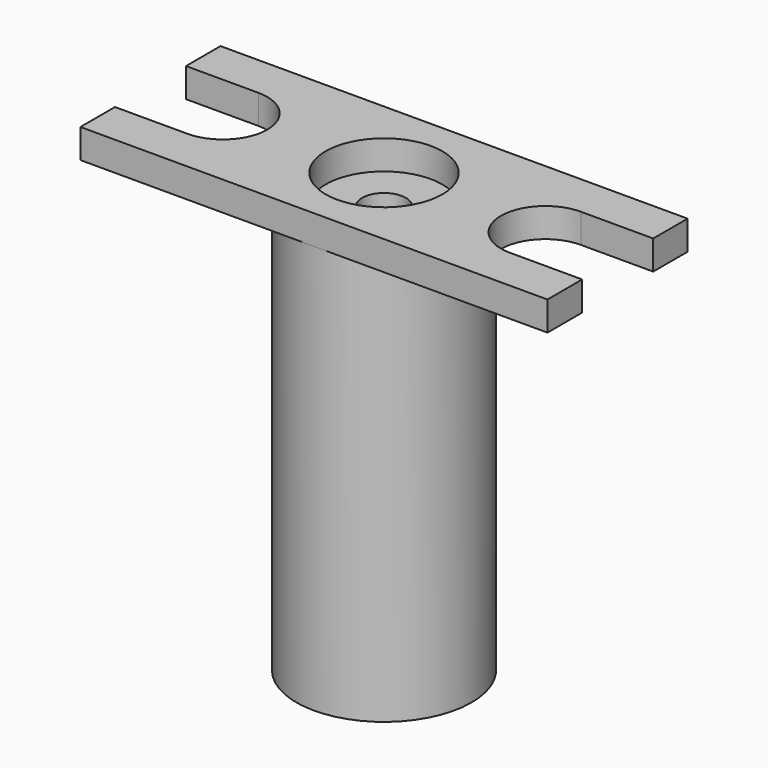
from build123d import *

# Parameters (mm, degrees)
F0_R        = 12.7
F1_DEPTH    = 6.35
F2_R        = 12.7
F3_DEPTH    = 63.5
F3_FACE_R   = 19.05
F3_FACE_R_2 = 12.7
F4_R        = 19.05
F4_R_2      = 4.7625
F5_DEPTH    = 25.4


with BuildPart() as f1:
    # F0 (on Top) → F1 (new body)
    with BuildSketch(Plane.XY):
        with BuildLine():
            Line((0, 9.398), (0, 0))
            Line((0, 0), (101.6, 0))
            Line((101.6, 0), (101.6, 9.4413837329))
            Line((101.6, 9.4413837329), (85.851973152, 9.4413837329))
            ThreePointArc((85.851973152, 9.4413837329), (76.199973152, 19.0933837329), (85.851973152, 28.7453837329))
            Line((85.851973152, 28.7453837329), (101.6, 28.7453837329))
            Line((101.6, 28.7453837329), (101.6, 38.1))
            Line((101.6, 38.1), (50.7999907375, 38.1))
            Line((50.7999907375, 38.1), (-1.85251e-05, 38.1))
            Line((-1.85251e-05, 38.1), (-1.85251e-05, 28.702))
            Line((-1.85251e-05, 28.702), (15.748, 28.702))
            ThreePointArc((15.748, 28.702), (25.4, 19.05), (15.748, 9.398))
            Line((15.748, 9.398), (0, 9.398))
        make_face()
        with Locations((50.8, 19.05)):
            Circle(F0_R, mode=Mode.SUBTRACT)
    extrude(amount=F1_DEPTH)

    # F2 (on face) → F3 (join)
    with BuildSketch(Plane(origin=(0, 0, 0), x_dir=(1, 0, 0), z_dir=(0, 0, -1))):
        with BuildLine():
            ThreePointArc((50.8, -38.1), (64.2703841816, -32.5203841816), (69.85, -19.05))
            ThreePointArc((69.85, -19.05), (64.2703841816, -5.5796158184), (50.8, 0))
            ThreePointArc((50.8, 0), (31.75, -19.05), (50.8, -38.1))
        make_face()
        with Locations((50.8, -19.05)):
            Circle(F2_R, mode=Mode.SUBTRACT)
    extrude(amount=F3_DEPTH)

    # F3_face (on face) + F4 (on Top) → F5 (join)
    with BuildSketch(Plane(origin=(50.8, 19.05, -63.5), x_dir=(1, 0, 0), z_dir=(0, 0, -1))):
        Circle(F3_FACE_R)
        Circle(F3_FACE_R_2, mode=Mode.SUBTRACT)
    with BuildSketch(Plane.XY):
        with Locations((50.8, 19.05)):
            Circle(F4_R)
        with Locations((50.8, 19.05)):
            Circle(F4_R_2, mode=Mode.SUBTRACT)
    extrude(amount=F5_DEPTH, dir=(0, 0, -1))


solid = f1.part
